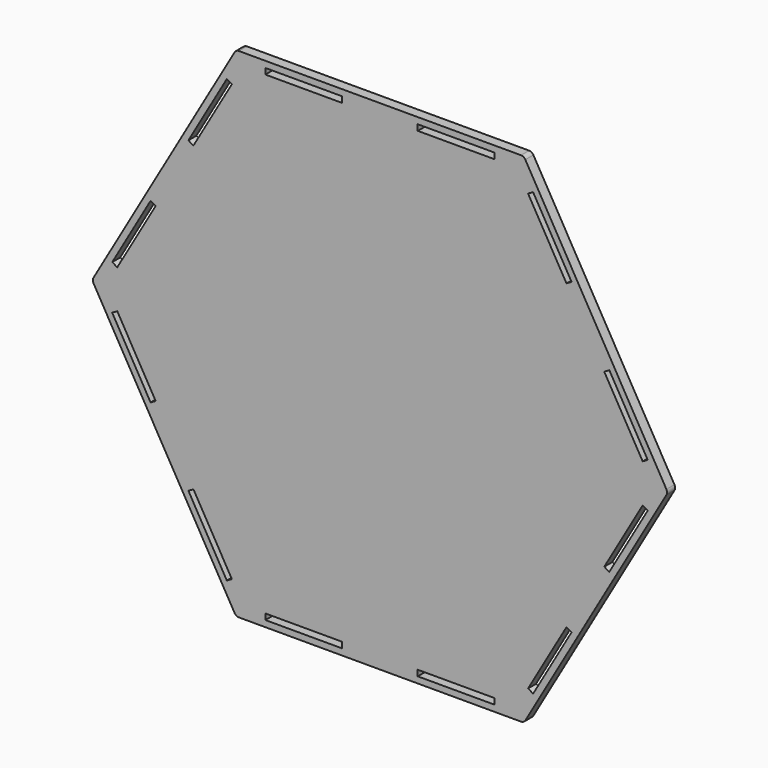
from build123d import *

# Parameters (mm, degrees)
F1_DEPTH        = 5.08
F2_W            = 38.7485525078
F2_H            = 2.9464
F3_DEPTH        = 5.08
F3_COPIES_COUNT = 6


# Not quite as in the source:
# - a pattern or mirror of a feature is missing from the dataset's text; its kind, count and spacing are read off the source's solid


with BuildPart() as f1:
    # F0 (on Front) → F1 (new body)
    with BuildSketch(Plane.XZ):
        with BuildLine():
            Line((71.1237796615, 125.73), (-71.1237796615, 125.73))
            ThreePointArc((-71.1237796615, 125.73), (-72.3937796615, 125.3897045256), (-73.3234841871, 124.46))
            Line((-73.3234841871, 124.46), (-144.4472638486, 1.27))
            ThreePointArc((-144.4472638486, 1.27), (-144.7875593229, 0), (-144.4472638486, -1.27))
            Line((-144.4472638486, -1.27), (-73.3234841871, -124.46))
            ThreePointArc((-73.3234841871, -124.46), (-72.3937796615, -125.3897045256), (-71.1237796615, -125.73))
            Line((-71.1237796615, -125.73), (71.1237796615, -125.73))
            ThreePointArc((71.1237796615, -125.73), (72.3937796615, -125.3897045256), (73.3234841871, -124.46))
            Line((73.3234841871, -124.46), (144.4472638486, -1.27))
            ThreePointArc((144.4472638486, -1.27), (144.7875593229, 0), (144.4472638486, 1.27))
            Line((144.4472638486, 1.27), (73.3234841871, 124.46))
            ThreePointArc((73.3234841871, 124.46), (72.3937796615, 125.3897045256), (71.1237796615, 125.73))
        make_face()
    extrude(amount=F1_DEPTH)

    # F2 (on face) → F3 (cut, through all)
    with BuildSketch(Plane.XZ.offset(5.08)):
        with Locations((-38.4242762539, 121.0818)):
            Rectangle(F2_W, F2_H)
        with Locations((38.4242762539, 121.0818)):
            Rectangle(F2_W, F2_H)
    f3 = extrude(amount=-F3_DEPTH, mode=Mode.SUBTRACT)

    # F3_copies: F3 ×6 about axis
    f3_copies_axis = Axis((0, 0, 0), (0, 1, 0))
    for i in range(1, F3_COPIES_COUNT):
        add(f3.rotate(f3_copies_axis, i * 360 / F3_COPIES_COUNT), mode=Mode.SUBTRACT)


solid = f1.part
